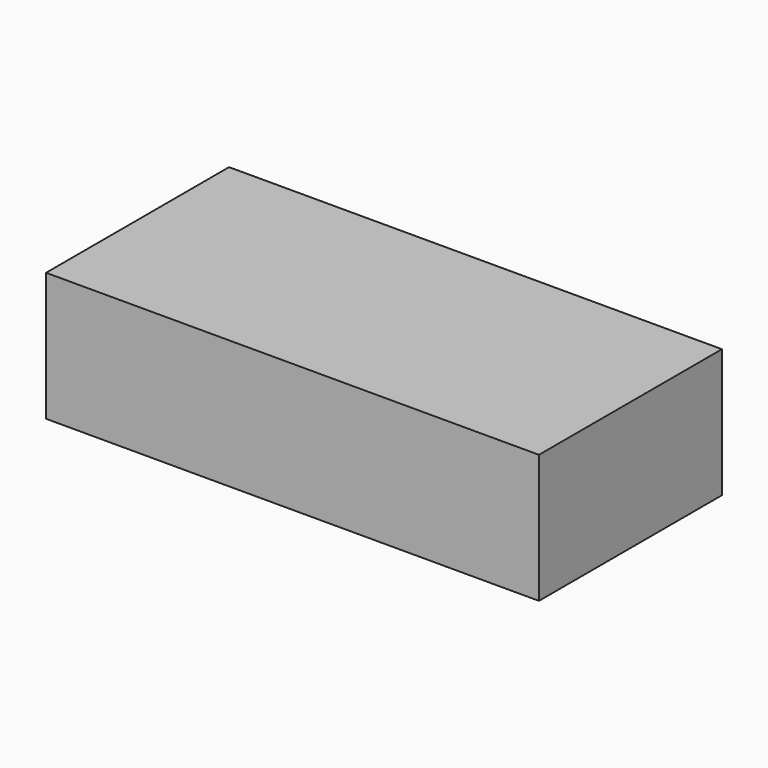
from build123d import *

# Parameters (mm, degrees)
F0_W     = 97.3527878523
F0_H     = 45.1786927879
F2_DEPTH = 25.4
F4_T     = -2.54


# Not quite as in the source:
# - the program builds the solid bodies; features that only make, move or delete a surface that nothing else refers to are left out


with BuildPart() as f2:
    # F0 (on Top) → F2 (new body)
    with BuildSketch(Plane.XY):
        with Locations((1.7488524318, 0)):
            Rectangle(F0_W, F0_H)
    extrude(amount=F2_DEPTH)

    # F4
    f4_openings = [f2.faces().sort_by_distance(p)[0] for p in [
        (1.748852, 0, 0),
    ]]
    offset(amount=F4_T, openings=f4_openings)


solid = f2.part
